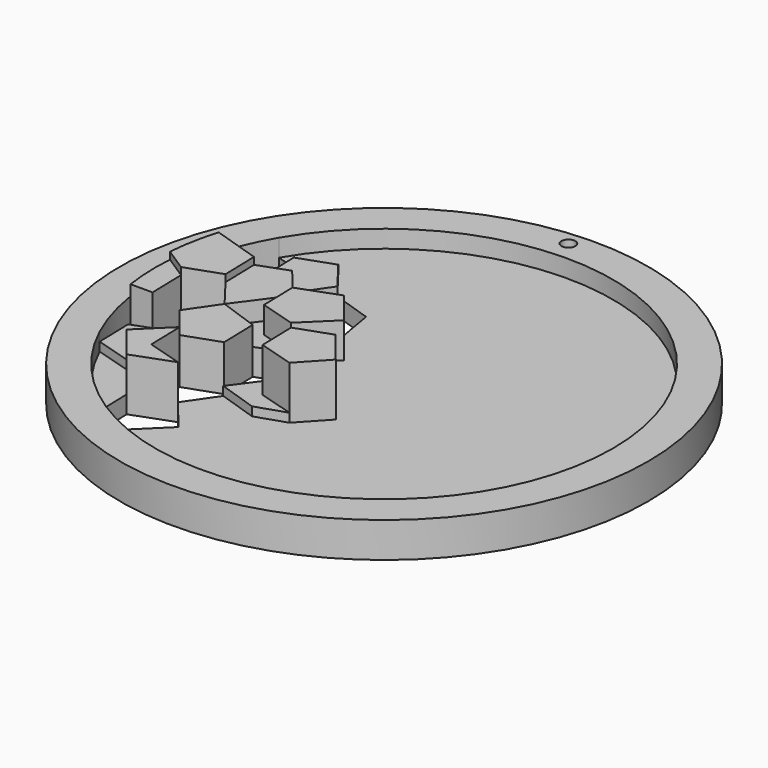
from build123d import *

# Parameters (mm, degrees)
F0_R     = 19.05
F1_DEPTH = 2.54
F2_DEPTH = 3.81
F3_DEPTH = 1.905
F4_DEPTH = 1.27
F5_DEPTH = 5.08
F6_DEPTH = 3.302
F8_D     = 1


# Not quite as in the source:
# - ends of sketch curves that miss each other by under 0.0002 mm in the source are joined


with BuildPart() as f1:
    # F0 (on Top) → F1 (new body)
    with BuildSketch(Plane.XY):
        with Locations((1.0659972724, 1.9032299986)):
            Circle(F0_R)
        with BuildLine():
            ThreePointArc((-13.1891179301, 10.2322029584), (5.3804003601, 17.8395415542), (17.5759972724, 1.9032299986))
            ThreePointArc((17.5759972724, 1.9032299986), (4.617214022, -14.2203229472), (-13.9163055256, -5.032957922))
            ThreePointArc((-13.9163055256, -5.032957922), (-14.7457872718, -2.8473036059), (-15.2582489012, -0.5664029427))
            ThreePointArc((-15.2582489012, -0.5664029427), (-15.4327964499, 1.2950312559), (-15.3957733388, 3.1642646312))
            ThreePointArc((-15.3957733388, 3.1642646312), (-15.1582970549, 4.9613950667), (-14.7252297792, 6.7216579795))
            ThreePointArc((-14.7252297792, 6.7216579795), (-14.0593672595, 8.5216473152), (-13.1891179301, 10.2322029584))
        make_face(mode=Mode.SUBTRACT)
    extrude(amount=F1_DEPTH)

    # F8 (through all)
    with Locations(Plane(origin=(0, 0, 0), x_dir=(1, 0, 0), z_dir=(0, 0, -1))):
        with Locations((0, -19.865270704)):
            Hole(F8_D / 2)


with BuildPart() as f2:
    # F0 (on Top) → F2 (new body)
    with BuildSketch(Plane.XY):
        Polygon((-4.4041624778, 5.1126668811), (-7.2693862148, 4.0531819443), (-7.2, 1.4), (-4.6552325034, 0.6461119018), (-2.5020106636, 2.7526948456), align=None)
    extrude(amount=F2_DEPTH)


with BuildPart() as f2b:
    # F0 (on Top) → F2, piece 2 (new body)
    with BuildSketch(Plane.XY):
        with BuildLine():
            Line((-11.3021234722, 5.6258294676), (-14.7252297792, 6.7216579795))
            ThreePointArc((-14.7252297792, 6.7216579795), (-15.1582970549, 4.9613950667), (-15.3957733388, 3.1642646312))
            Line((-15.3957733388, 3.1642646312), (-13.7346217148, 2.0867790016))
            Line((-13.7346217148, 2.0867790016), (-11.2327372573, 2.9726475233))
            Line((-11.2327372573, 2.9726475233), (-11.3021234722, 5.6258294676))
        make_face()
    extrude(amount=F2_DEPTH)


with BuildPart() as f2c:
    # F0 (on Top) → F2, piece 3 (new body)
    with BuildSketch(Plane.XY):
        Polygon((-9.2183161892, -3.6802630764), (-11.371538029, -5.7868460202), (-9.4693862148, -8.1468180557), (-6.6041624778, -7.0873331189), (-9.1489299744, -6.3334450207), align=None)
    extrude(amount=F2_DEPTH)


with BuildPart() as f3:
    # F0 (on Top) → F3 (new body)
    with BuildSketch(Plane.XY):
        Polygon((-7.2693862148, 4.0531819443), (-9.6171014119, 0.866962435), (-6.7858179466, -0.1412126104), (-4.6552325034, 0.6461119018), (-7.2, 1.4), align=None)
    extrude(amount=F3_DEPTH)


with BuildPart() as f3b:
    # F0 (on Top) → F3, piece 2 (new body)
    with BuildSketch(Plane.XY):
        Polygon((-13.9856917404, -2.3797759777), (-13.9163055256, -5.032957922), (-11.371538029, -5.7868460202), (-9.2183161892, -3.6802630764), (-11.1204680034, -1.3202910409), align=None)
    extrude(amount=F3_DEPTH)


with BuildPart() as f3c:
    # F0 (on Top) → F3, piece 3 (new body)
    with BuildSketch(Plane.XY):
        Polygon((-9.2834670883, 10.7059926791), (-11.7853515458, 9.8201241574), (-11.7159653309, 7.1669422131), (-9.171538029, 6.4131539798), (-7.6681714375, 8.6004074557), (-7.6678349877, 8.6002962598), align=None)
    extrude(amount=F3_DEPTH)


with BuildPart() as f3d:
    # F0 (on Top) → F3, piece 4 (new body)
    with BuildSketch(Plane.XY):
        Polygon((-2.7530806892, -1.7138601337), (-5.1007958863, -4.900079643), (-2.2774721557, -5.8331822828), (-0.1389269778, -5.1209301762), (-2.6836944744, -4.367042078), align=None)
    extrude(amount=F3_DEPTH)


with BuildPart() as f4:
    # F0 (on Top) → F4 (new body)
    with BuildSketch(Plane.XY):
        with BuildLine():
            ThreePointArc((-13.9163055256, -5.032957922), (4.617214022, -14.2203229472), (17.5759972724, 1.9032299986))
            ThreePointArc((17.5759972724, 1.9032299986), (5.3804003601, 17.8395415542), (-13.1891179301, 10.2322029584))
            Line((-13.1891179301, 10.2322029584), (-11.7853515458, 9.8201241574))
            Line((-11.7853515458, 9.8201241574), (-9.2834670883, 10.7059926791))
            Line((-9.2834670883, 10.7059926791), (-7.6678312428, 8.6003075908))
            Line((-7.6678312428, 8.6003075908), (-4.8448477069, 7.6673048159))
            Line((-4.8448477069, 7.6673048159), (-4.4041624778, 5.1126668811))
            Line((-4.4041624778, 5.1126668811), (-2.5020106636, 2.7526948456))
            Line((-2.5020106636, 2.7526948456), (-4.6552325034, 0.6461119018))
            Line((-4.6552325034, 0.6461119018), (-2.7530806892, -1.7138601337))
            Line((-2.7530806892, -1.7138601337), (-0.2511962318, -0.827991612))
            Line((-0.2511962318, -0.827991612), (1.6509555824, -3.1879636476))
            Line((1.6509555824, -3.1879636476), (-0.1389269778, -5.1209301762))
            Line((-0.1389269778, -5.1209301762), (-2.2774721557, -5.8331822828))
            Line((-2.2774721557, -5.8331822828), (-5.1007958863, -4.900079643))
            Line((-5.1007958863, -4.900079643), (-6.6041624778, -7.0873331189))
            Line((-6.6041624778, -7.0873331189), (-4.7020106636, -9.4473051544))
            Line((-4.7020106636, -9.4473051544), (-6.8552325034, -11.5538880982))
            Line((-6.8552325034, -11.5538880982), (-9.4, -10.8))
            Line((-9.4, -10.8), (-9.4693862148, -8.1468180557))
            Line((-9.4693862148, -8.1468180557), (-11.371538029, -5.7868460202))
            Line((-11.371538029, -5.7868460202), (-13.9163055256, -5.032957922))
        make_face()
    extrude(amount=F4_DEPTH)


with BuildPart() as f5:
    # F0 (on Top) → F5 (new body)
    with BuildSketch(Plane.XY):
        Polygon((-0.2511962318, -0.827991612), (-2.7530806892, -1.7138601337), (-2.6836944744, -4.367042078), (-0.1389269778, -5.1209301762), (1.6509555824, -3.1879636476), align=None)
    extrude(amount=F5_DEPTH)


with BuildPart() as f6:
    # F0 (on Top) → F6 (new body)
    with BuildSketch(Plane.XY):
        Polygon((-9.171538029, 6.4131539798), (-11.3021234722, 5.6258294676), (-11.2327372573, 2.9726475233), (-9.6171014119, 0.866962435), (-7.2693862148, 4.0531819443), align=None)
    extrude(amount=F6_DEPTH)


with BuildPart() as f6b:
    # F0 (on Top) → F6, piece 2 (new body)
    with BuildSketch(Plane.XY):
        Polygon((-11.1204680034, -1.3202910409), (-9.2183161892, -3.6802630764), (-6.7164317317, -2.7943945547), (-6.7858179466, -0.1412126104), (-9.6171014119, 0.866962435), align=None)
    extrude(amount=F6_DEPTH)


with BuildPart() as f6c:
    # F0 (on Top) → F6, piece 3 (new body)
    with BuildSketch(Plane.XY):
        with BuildLine():
            ThreePointArc((-15.3957733388, 3.1642646312), (-15.4327964499, 1.2950312559), (-15.2582489012, -0.5664029427))
            Line((-15.2582489012, -0.5664029427), (-13.6652355, -0.5664029427))
            Line((-13.6652355, -0.5664029427), (-13.7346217148, 2.0867790016))
            Line((-13.7346217148, 2.0867790016), (-15.3957733388, 3.1642646312))
        make_face()
    extrude(amount=F6_DEPTH)


solid = Compound([f1.part, f2.part, f2b.part, f2c.part, f3.part, f3b.part, f3c.part, f3d.part, f4.part, f5.part, f6.part, f6b.part, f6c.part])
